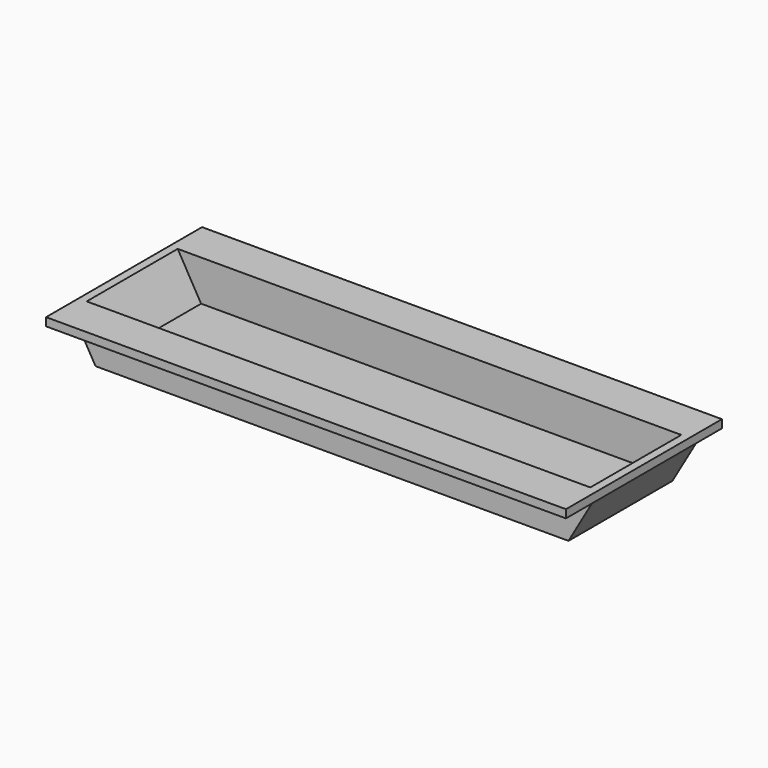
from build123d import *

# Parameters (mm, degrees)
F0_W      = 101.6
F0_H      = 38.1
F1_DEPTH  = 203.2
F3_T      = -6.35
F2_W      = 406.4
F2_H      = 6.35
F4_DEPTH  = 25.4
F5_W      = 406.4
F5_H      = 6.35
F6_DEPTH  = 25.4
F8_DEPTH  = 88.9
F10_DEPTH = 141.224


# Not quite as in the source:
# - a pattern or mirror of a feature is missing from the dataset's text; its kind, count and spacing are read off the source's solid


with BuildPart() as f1:
    # F0 (on Right) → F1 (new body, symmetric)
    with BuildSketch(Plane.YZ):
        with Locations((50.8, 19.05)):
            Rectangle(F0_W, F0_H)
    extrude(amount=F1_DEPTH, both=True)

    # F3
    f3_openings = [f1.faces().sort_by_distance(p)[0] for p in [
        (0, 50.8, 38.1),
    ]]
    offset(amount=F3_T, openings=f3_openings)

    # F2 (on face) → F4 (join)
    with BuildSketch(Plane.XZ):
        with Locations((0, 34.925)):
            Rectangle(F2_W, F2_H)
    extrude(amount=F4_DEPTH)

    # F5 (on face) → F6 (join)
    with BuildSketch(Plane(origin=(0, 101.6, 0), x_dir=(-1, 0, 0), z_dir=(0, 1, 0))):
        with Locations((0, 34.925)):
            Rectangle(F5_W, F5_H)
    extrude(amount=F6_DEPTH)

    # F7 (on face) → F8 (join, through all)
    with BuildSketch(Plane(origin=(0, 6.35, 0), x_dir=(-1, 0, 0), z_dir=(0, 1, 0))):
        Polygon((196.85, 6.35), (196.85, 38.1), (178.5191289532, 6.35), align=None)
    f8 = extrude(amount=F8_DEPTH)

    # F8_copies: F8 across plane
    add(f8.mirror(Plane(origin=(0, 0, 0), x_dir=(0, 0, 1), z_dir=(1, 0, 0))))

    # F9 (on Front) → F10 (cut)
    with BuildSketch(Plane.XZ):
        Polygon((-184.8691289532, 0), (-203.2, 31.75), (-203.2, 0), align=None)
    f10 = extrude(amount=-F10_DEPTH, mode=Mode.SUBTRACT)

    # F10_copies: F10 across plane
    add(f10.mirror(Plane(origin=(0, 0, 0), x_dir=(0, 0, 1), z_dir=(1, 0, 0))), mode=Mode.SUBTRACT)


solid = f1.part
